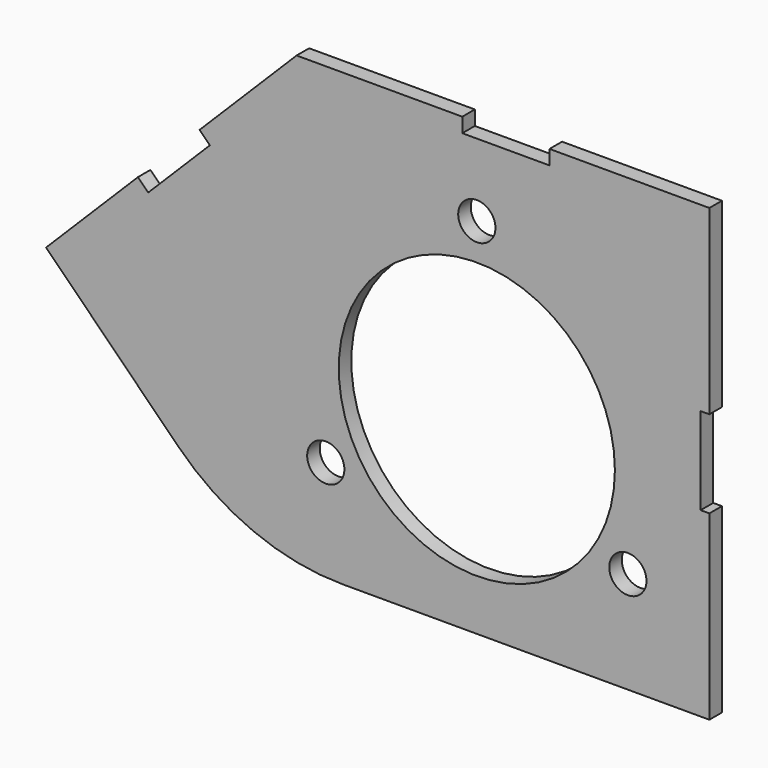
from build123d import *

# Parameters (mm, degrees)
F0_R     = 4.064
F0_R_2   = 30.1625
F1_DEPTH = 3.429


# Not quite as in the source:
# - ends of sketch curves that miss each other by under 0.0002 mm in the source are joined


with BuildPart() as f1:
    # F0 (on Front) → F1 (new body)
    with BuildSketch(Plane.XZ):
        with BuildLine():
            Line((-405.5923562, 237.0029296), (-419.0627382, 223.5325476))
            Line((-419.0627382, 223.5325476), (-421.3077934, 225.7776028))
            Line((-421.3077934, 225.7776028), (-441.368434, 205.7169622))
            Line((-441.368434, 205.7169622), (-412.5468254, 176.895379))
            ThreePointArc((-412.5468254, 176.895379), (-396.0661335641, 165.8833089484), (-376.6258152, 162.0163892))
            Line((-376.6258152, 162.0163892), (-296.474007, 162.0163892))
            Line((-296.474007, 162.0163892), (-296.474007, 201.7038892))
            Line((-296.474007, 201.7038892), (-298.379007, 201.7038892))
            Line((-298.379007, 201.7038892), (-298.379007, 220.7538892))
            Line((-298.379007, 220.7538892), (-296.474007, 220.7538892))
            Line((-296.474007, 220.7538892), (-296.474007, 260.4413892))
            Line((-296.474007, 260.4413892), (-331.399007, 260.4413892))
            Line((-331.399007, 260.4413892), (-331.399007, 257.2663892))
            Line((-331.399007, 257.2663892), (-350.449007, 257.2663892))
            Line((-350.449007, 257.2663892), (-350.449007, 260.4413892))
            Line((-350.449007, 260.4413892), (-386.644007, 260.4413892))
            Line((-386.644007, 260.4413892), (-407.8374114, 239.2479848))
            Line((-407.8374114, 239.2479848), (-405.5923562, 237.0029296))
        make_face()
        with Locations((-380.2695722, 184.2413892)):
            Circle(F0_R, mode=Mode.SUBTRACT)
        with Locations((-314.2784418, 184.2413892)):
            Circle(F0_R, mode=Mode.SUBTRACT)
        with Locations((-347.274007, 203.2913892)):
            Circle(F0_R_2, mode=Mode.SUBTRACT)
        with Locations((-347.274007, 241.3913892)):
            Circle(F0_R, mode=Mode.SUBTRACT)
    extrude(amount=F1_DEPTH)


solid = f1.part
